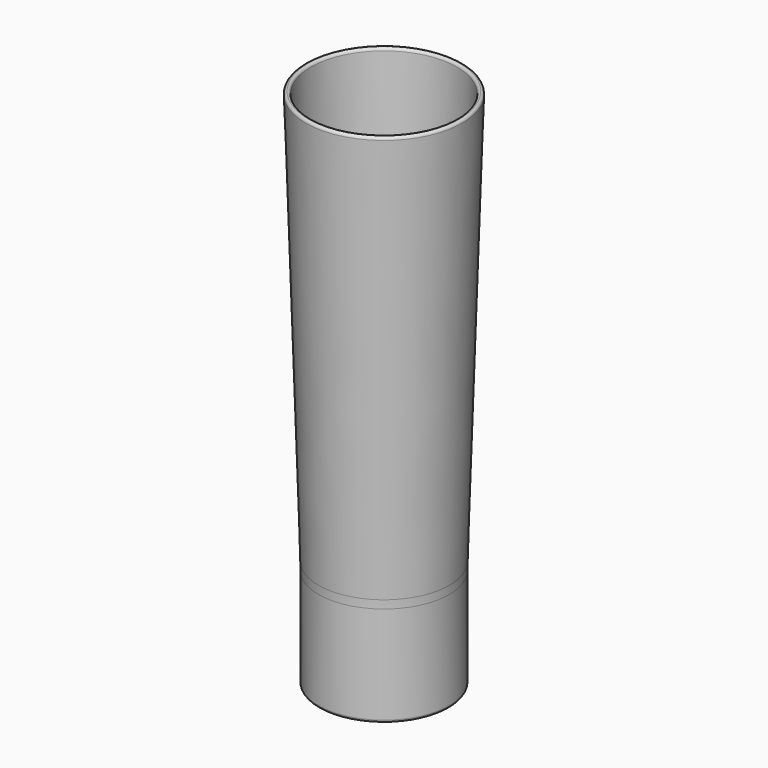
from build123d import *

# Parameters (mm, degrees)
F3_R = 0.99999


# Not quite as in the source:
# - a fillet or chamfer that OpenCascade refuses, or shapes differently, is made with other operations: its cross-section is extruded or revolved along the edge and cut away or added
# - a fillet or chamfer is up to 0.001 mm smaller than in the source, because OpenCascade refuses the exact size


with BuildPart() as f1:
    # F0 (on Front) → F1 (revolve)
    with BuildSketch(Plane.XZ):
        Polygon((-23, -114.1254802332), (-27.9990236758, 45.8432773924), (-30, 45.8432773924), (-25, -114.1567226076), (-25, -154.1567226076), (-23, -154.1567226076), align=None)
    revolve(axis=Axis((0, 0, -54.1567226076), (0, 0, 1)))

    # F2: fillet of radius 100 on 2 edges, made by hand

    # F2_s1 → F2_t2 (revolve)
    with BuildSketch(Plane.XZ):
        with BuildLine():
            ThreePointArc((-25.0487923913, -112.5953660862), (-25.0121988419, -114.1569131679), (-25, -115.718841324))
            Line((-25, -115.718841324), (-25, -114.1567226076))
            Line((-25, -114.1567226076), (-25.0487923913, -112.5953660862))
        make_face()
    revolve(axis=Axis((0, 0, -114.1567226076), (0, 0, 1)))

    # F2_s3 → F2_t4 (revolve, cut)
    with BuildSketch(Plane.XZ):
        with BuildLine():
            ThreePointArc((-23.0487923913, -112.5641237119), (-23.0121988419, -114.1256707936), (-23, -115.6875989497))
            Line((-23, -115.6875989497), (-23, -114.1254802332))
            Line((-23, -114.1254802332), (-23.0487923913, -112.5641237119))
        make_face()
    revolve(axis=Axis((0, 0, -114.1254802332), (0, 0, 1)), mode=Mode.SUBTRACT)

    # F3 (radius 1 in the source; OpenCascade refuses exactly that, so slightly less here)
    f3_edges = [f1.edges().sort_by_distance(p)[0] for p in [
        (27.999024, 0, 45.843277),
        (30, 0, 45.843277),
        (25, 0, -154.156723),
        (23, 0, -154.156723),
    ]]
    fillet(f3_edges, radius=F3_R)


solid = f1.part
